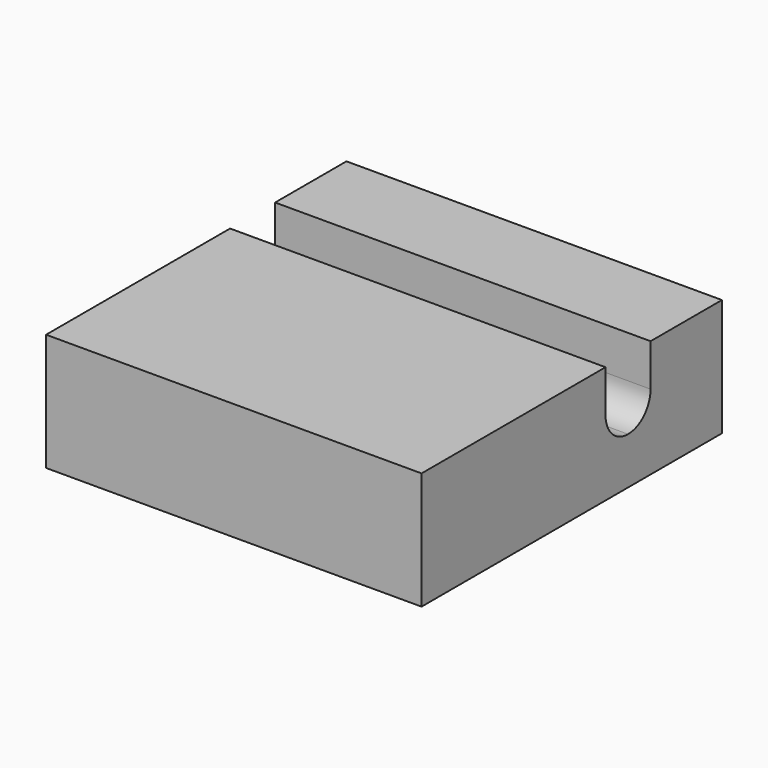
from build123d import *

# Parameters (mm, degrees)
F0_W     = 80
F0_H     = 80
F1_DEPTH = 25
F2_W     = 80
F2_H     = 12
F3_DEPTH = 15
F4_R     = 5.99999


# Not quite as in the source:
# - a fillet or chamfer is up to 0.001 mm smaller than in the source, because OpenCascade refuses the exact size


with BuildPart() as f1:
    # F0 (on Top) → F1 (new body)
    with BuildSketch(Plane.XY):
        Rectangle(F0_W, F0_H)
    extrude(amount=F1_DEPTH)

    # F2 (on face) → F3 (cut)
    with BuildSketch(Plane.XY.offset(25)):
        with Locations((0, 15)):
            Rectangle(F2_W, F2_H)
    extrude(amount=-F3_DEPTH, mode=Mode.SUBTRACT)

    # F4 (radius 6 in the source; OpenCascade refuses exactly that, so slightly less here)
    f4_edges = [f1.edges().sort_by_distance(p)[0] for p in [
        (0, 9, 10),
        (0, 21, 10),
    ]]
    fillet(f4_edges, radius=F4_R)


solid = f1.part
